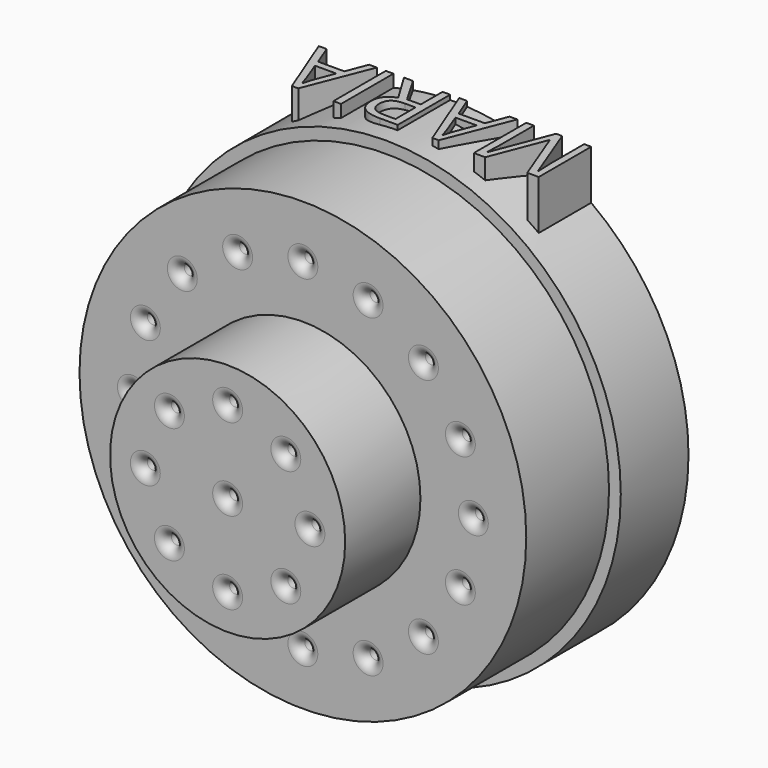
from build123d import *

# Parameters (mm, degrees)
F0_R         = 50
F1_DEPTH     = 18
F2_R         = 47.5
F2_R_2       = 1.18
F3_DEPTH     = 22
F4_R         = 25
F4_R_2       = 1.18
F5_DEPTH     = 20
F6_TEXT_SIZE = 19.5245731447
F7_DEPTH     = 51
F8_R         = 2
F9_R         = 47.5189367606
F10_DEPTH    = 16.7


# Not quite as in the source:
# - Text() gives the source's letters only with a copy of the font that has no kerning and outlines rounded to 1/6400 em; it was checked with that copy


with BuildPart() as f1:
    # F0 (on Front) → F1 (new body)
    with BuildSketch(Plane.XZ):
        Circle(F0_R)
    extrude(amount=F1_DEPTH)

    # F2 (on face) → F3 (join)
    with BuildSketch(Plane.XZ.offset(18)):
        Circle(F2_R)
        with Locations((-25.632620818, -25.632620818)):
            Circle(F2_R_2, mode=Mode.SUBTRACT)
        with Locations((-13.8722744232, -33.4906330535)):
            Circle(F2_R_2, mode=Mode.SUBTRACT)
        with Locations((-33.4906330535, -13.8722744232)):
            Circle(F2_R_2, mode=Mode.SUBTRACT)
        with Locations((0, -36.25)):
            Circle(F2_R_2, mode=Mode.SUBTRACT)
        with Locations((13.8722744232, -33.4906330535)):
            Circle(F2_R_2, mode=Mode.SUBTRACT)
        with Locations((25.632620818, -25.632620818)):
            Circle(F2_R_2, mode=Mode.SUBTRACT)
        with Locations((33.4906330535, -13.8722744232)):
            Circle(F2_R_2, mode=Mode.SUBTRACT)
        with Locations((-36.25, 0)):
            Circle(F2_R_2, mode=Mode.SUBTRACT)
        with Locations((-33.4906330535, 13.8722744232)):
            Circle(F2_R_2, mode=Mode.SUBTRACT)
        with Locations((-25.632620818, 25.632620818)):
            Circle(F2_R_2, mode=Mode.SUBTRACT)
        with Locations((-13.8722744232, 33.4906330535)):
            Circle(F2_R_2, mode=Mode.SUBTRACT)
        with Locations((36.25, 0)):
            Circle(F2_R_2, mode=Mode.SUBTRACT)
        with Locations((33.4906330535, 13.8722744232)):
            Circle(F2_R_2, mode=Mode.SUBTRACT)
        with Locations((0, 36.25)):
            Circle(F2_R_2, mode=Mode.SUBTRACT)
        with Locations((13.8722744232, 33.4906330535)):
            Circle(F2_R_2, mode=Mode.SUBTRACT)
        with Locations((25.632620818, 25.632620818)):
            Circle(F2_R_2, mode=Mode.SUBTRACT)
    extrude(amount=F3_DEPTH)

    # F4 (on face) → F5 (join)
    with BuildSketch(Plane.XZ.offset(40)):
        Circle(F4_R)
        with Locations((-12.3743686708, -12.3743686708)):
            Circle(F4_R_2, mode=Mode.SUBTRACT)
        with Locations((0, -17.5)):
            Circle(F4_R_2, mode=Mode.SUBTRACT)
        with Locations((12.3743686708, -12.3743686708)):
            Circle(F4_R_2, mode=Mode.SUBTRACT)
        with Locations((-17.5, 0)):
            Circle(F4_R_2, mode=Mode.SUBTRACT)
        with Locations((-12.3743686708, 12.3743686708)):
            Circle(F4_R_2, mode=Mode.SUBTRACT)
        Circle(F4_R_2, mode=Mode.SUBTRACT)
        with Locations((17.5, 0)):
            Circle(F4_R_2, mode=Mode.SUBTRACT)
        with Locations((0, 17.5)):
            Circle(F4_R_2, mode=Mode.SUBTRACT)
        with Locations((12.3743686708, 12.3743686708)):
            Circle(F4_R_2, mode=Mode.SUBTRACT)
    extrude(amount=F5_DEPTH)

    # F6 (on Top) → F7 (join)
    with BuildSketch(Plane.XY):
        with Locations(Location((31.2211532146, 0), (0, 0, -180))):
            Text('MARIA', F6_TEXT_SIZE, font='Open Sans', text_align=(TextAlign.LEFT, TextAlign.BOTTOM))
    extrude(amount=F7_DEPTH)

    # F8
    f8_edges = [f1.edges().sort_by_distance(p)[0] for p in [
        (-34.670633, -40, 13.872274),
        (-37.43, -40, 0),
        (-34.670633, -40, -13.872274),
        (-26.812621, -40, -25.632621),
        (-15.052274, -40, -33.490633),
        (-1.18, -40, -36.25),
        (12.692274, -40, -33.490633),
        (24.452621, -40, -25.632621),
        (32.310633, -40, -13.872274),
        (35.07, -40, 0),
        (32.310633, -40, 13.872274),
        (24.452621, -40, 25.632621),
        (12.692274, -40, 33.490633),
        (-1.18, -40, 36.25),
        (-15.052274, -40, 33.490633),
        (-26.812621, -40, 25.632621),
        (-13.554369, -60, 12.374369),
        (-18.68, -60, 0),
        (-13.554369, -60, -12.374369),
        (-1.18, -60, -17.5),
        (11.194369, -60, -12.374369),
        (16.32, -60, 0),
        (11.194369, -60, 12.374369),
        (-1.18, -60, 17.5),
        (-1.18, -60, 0),
    ]]
    fillet(f8_edges, radius=F8_R)

    # F9 (on Front) → F10 (cut)
    with BuildSketch(Plane.XZ):
        Circle(F9_R)
    extrude(amount=F10_DEPTH, mode=Mode.SUBTRACT)


solid = f1.part
